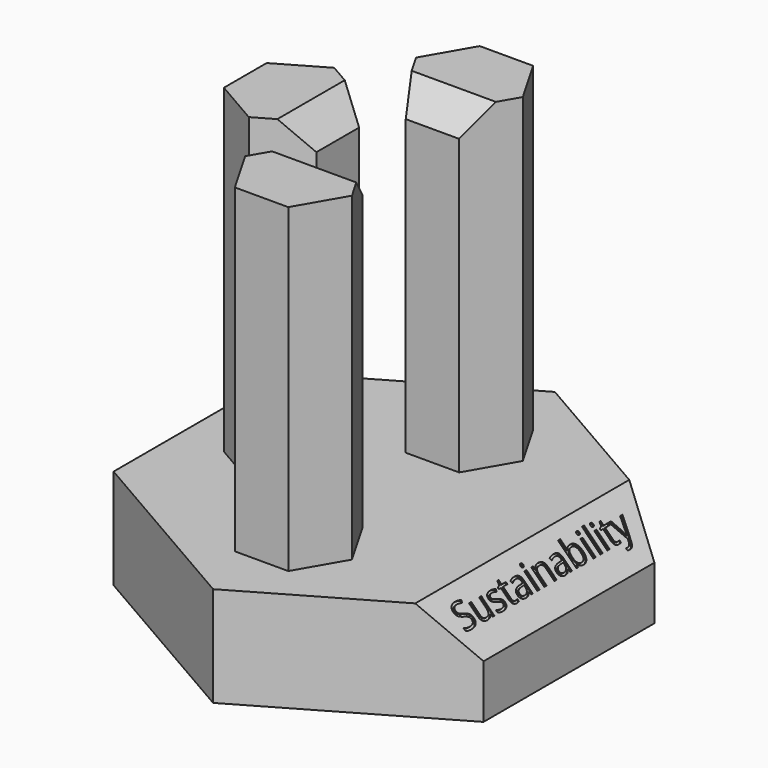
from build123d import *

# Parameters (mm, degrees)
F1_DEPTH     = 63.5
F3_DEPTH     = 127
F4_SIZE      = 88.9
F6_DEPTH     = 609.6
F7_DEPTH     = 609.6
F8_SIZE      = 50.8
F9_TEXT_SIZE = 65.5566477631
F10_DEPTH    = 2.54


# Not quite as in the source:
# - a feature names something its author has since deleted; it is built from what else it names
# - Text() gives the source's letters only with a copy of the font that has no kerning and outlines rounded to 1/6400 em; it was checked with that copy


with BuildPart() as f1:
    # F0 (on Top) → F1 (new body)
    with BuildSketch(Plane.XY):
        Polygon((351.952724098, -203.2), (351.952724098, 203.2), (0, 406.4), (-351.952724098, 203.2), (-351.952724098, -203.2), (0, -406.4), align=None)
    extrude(amount=F1_DEPTH)

    # F2 (on face) → F3 (join)
    with BuildSketch(Plane(origin=(0, 0, 0), x_dir=(1, 0, 0), z_dir=(0, 0, -1))):
        Polygon((351.952724098, -203.2), (351.952724098, 203.2), (0, 406.4), (-351.952724098, 203.2), (-351.952724098, -203.2), (0, -406.4), align=None)
    extrude(amount=F3_DEPTH)

    # F4
    f4_edges = [f1.edges().sort_by_distance(p)[0] for p in [
        (351.952724, 0, 63.5),
    ]]
    chamfer(f4_edges, length=F4_SIZE)

    # F5 (on face) → F6 (join)
    with BuildSketch(Plane.XY.offset(63.5)):
        Polygon((-175.976362049, 0), (-263.9645430735, 0), (-263.9645430735, -50.8), (-175.976362049, -101.6), (-87.9881810245, -50.8), (-87.9881810245, 0), align=None)
        Polygon((-263.9645430735, 50.8), (-263.9645430735, 0), (-175.976362049, 0), (-87.9881810245, 0), (-87.9881810245, 50.8), (-175.976362049, 101.6), align=None)
    extrude(amount=F6_DEPTH)

    # F5 (on face) → F7 (join)
    with BuildSketch(Plane.XY.offset(63.5)):
        Polygon((-50.8, -291.1881810245), (0, -291.1881810245), (0, -203.2), (0, -115.2118189755), (-50.8, -115.2118189755), (-101.6, -203.2), align=None)
        Polygon((0, -203.2), (0, -291.1881810245), (50.8, -291.1881810245), (101.6, -203.2), (50.8, -115.2118189755), (0, -115.2118189755), align=None)
        Polygon((-87.9881810245, -50.8), (-87.9881810245, 0), (-175.976362049, 0), (-263.9645430735, 0), (-263.9645430735, -50.8), (-175.976362049, -101.6), align=None)
        Polygon((-175.976362049, 0), (-87.9881810245, 0), (-87.9881810245, 50.8), (-175.976362049, 101.6), (-263.9645430735, 50.8), (-263.9645430735, 0), align=None)
        Polygon((-50.8, 115.2118189755), (0, 115.2118189755), (0, 203.2), (0, 291.1881810245), (-50.8, 291.1881810245), (-101.6, 203.2), align=None)
        Polygon((0, 203.2), (0, 115.2118189755), (50.8, 115.2118189755), (101.6, 203.2), (50.8, 291.1881810245), (0, 291.1881810245), align=None)
    extrude(amount=F7_DEPTH)

    # F8
    f8_edges = [f1.edges().sort_by_distance(p)[0] for p in [
        (0, -115.211819, 673.1),
        (-87.988181, 0, 673.1),
        (0, 115.211819, 673.1),
    ]]
    chamfer(f8_edges, length=F8_SIZE)

    # F9 (on face) → F10 (cut)
    with BuildSketch(Plane(origin=(163.276362049, 0, 163.276362049), x_dir=(0, 1, 0), z_dir=(0.7071067812, 0, 0.7071067812))):
        with Locations((-203.181561069, -216.0286701089)):
            Text('Sustainability', F9_TEXT_SIZE, font='Open Sans', text_align=(TextAlign.LEFT, TextAlign.BOTTOM))
    extrude(amount=-F10_DEPTH, mode=Mode.SUBTRACT)


solid = f1.part
